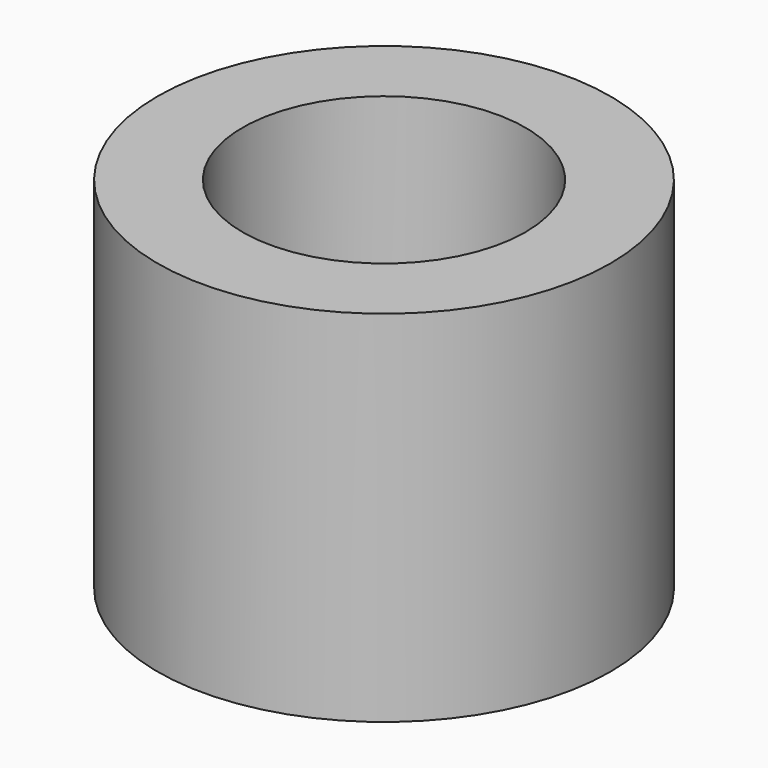
from build123d import *

# Parameters (mm, degrees)
F0_R     = 4
F0_R_2   = 2.5
F1_DEPTH = 6.35


# Not quite as in the source:
# - a length typed as a fraction of an inch, garbled in the dataset ("3 / 203.2 mm" for 3/8 in), is restored


with BuildPart() as f1:
    # F0 (on Top) → F1 (new body)
    with BuildSketch(Plane.XY):
        Circle(F0_R)
        Circle(F0_R_2, mode=Mode.SUBTRACT)
    extrude(amount=F1_DEPTH)


solid = f1.part
